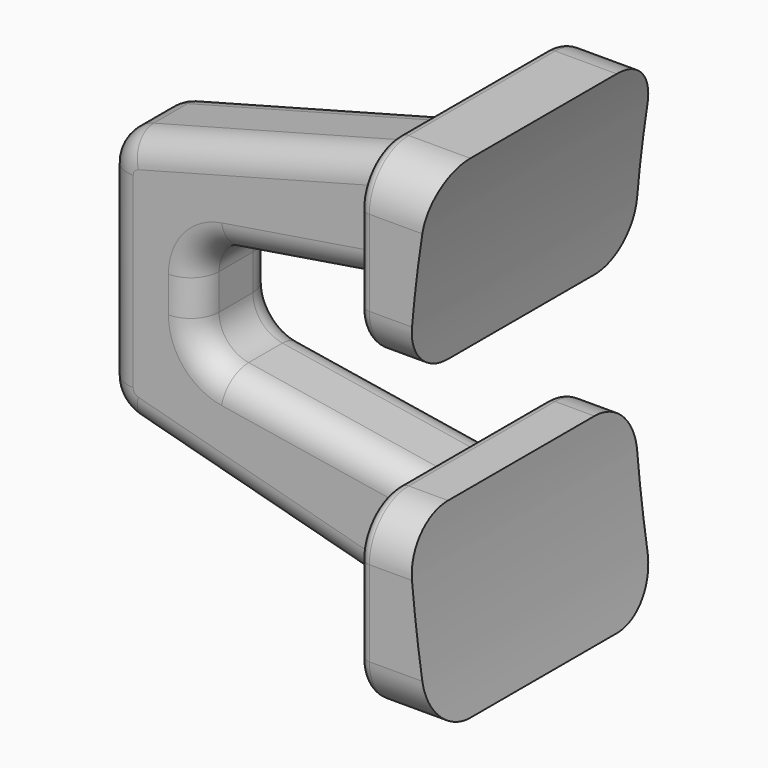
from build123d import *

# Parameters (mm, degrees)
F1_DEPTH = 1.778
F3_DEPTH = 5.08
F4_R     = 1.778
F5_R     = 0.381
F6_R     = 1.27
F7_R     = 1.016
F8_R     = 0.254


# Not quite as in the source:
# - a feature names something its author has since deleted; it is built from what else it names


with BuildPart() as f1:
    # F0 (on Front) → F1 (new body, symmetric)
    with BuildSketch(Plane.XZ):
        with BuildLine():
            Line((-31.496, -8.89), (-28.8890805669, -8.89))
            ThreePointArc((-28.8890805669, -8.89), (-29.4117334596, -5.5835621932), (-29.6945393604, -2.2480385704))
            Line((-29.6945393604, -2.2480385704), (-31.496, -2.2480385704))
            Line((-31.496, -2.2480385704), (-31.496, -3.0988187389))
            Line((-31.496, -3.0988187389), (-39.9942283773, -1.7265919268))
            Line((-39.9942283773, -1.7265919268), (-39.9942283773, 0))
            Line((-39.9942283773, 0), (-39.9942283773, 1.7265919268))
            Line((-39.9942283773, 1.7265919268), (-31.496, 3.0988187389))
            Line((-31.496, 3.0988187389), (-31.496, 2.2480385704))
            Line((-31.496, 2.2480385704), (-29.6945393604, 2.2480385704))
            ThreePointArc((-29.6945393604, 2.2480385704), (-29.4117334596, 5.5835621932), (-28.8890805669, 8.89))
            Line((-28.8890805669, 8.89), (-31.496, 8.89))
            Line((-31.496, 8.89), (-31.496, 7.4847033247))
            Line((-31.496, 7.4847033247), (-43.2962283773, 4.3461126307))
            Line((-43.2962283773, 4.3461126307), (-43.2962283773, 0))
            Line((-43.2962283773, 0), (-43.2962283773, -4.3461126307))
            Line((-43.2962283773, -4.3461126307), (-31.496, -7.4847033247))
            Line((-31.496, -7.4847033247), (-31.496, -8.89))
        make_face()
    extrude(amount=F1_DEPTH, both=True)

    # F2 (on Front) → F3 (join, symmetric)
    with BuildSketch(Plane.XZ):
        with BuildLine():
            Line((-28.8890805669, 8.89), (-31.496, 8.89))
            Line((-31.496, 8.89), (-31.496, 2.2480385704))
            Line((-31.496, 2.2480385704), (-29.6945393604, 2.2480385704))
            ThreePointArc((-29.6945393604, 2.2480385704), (-29.4117334596, 5.5835621932), (-28.8890805669, 8.89))
        make_face()
        with BuildLine():
            Line((-31.496, -2.2480385704), (-31.496, -8.89))
            Line((-31.496, -8.89), (-28.8890805669, -8.89))
            ThreePointArc((-28.8890805669, -8.89), (-29.4117334596, -5.5835621932), (-29.6945393604, -2.2480385704))
            Line((-29.6945393604, -2.2480385704), (-31.496, -2.2480385704))
        make_face()
    extrude(amount=F3_DEPTH, both=True)

    # F4
    f4_edges = [f1.edges().sort_by_distance(p)[0] for p in [
        (-30.19254, -5.08, 8.89),
        (-30.19254, 5.08, 8.89),
        (-30.19254, 5.08, -8.89),
        (-30.19254, -5.08, -8.89),
        (-30.59527, -5.08, -2.248039),
        (-30.59527, -5.08, 2.248039),
        (-30.59527, 5.08, -2.248039),
        (-30.59527, 5.08, 2.248039),
    ]]
    fillet(f4_edges, radius=F4_R)

    # F5
    f5_edges = [f1.edges().sort_by_distance(p)[0] for p in [
        (-31.496, 5.08, 5.569019),
        (-31.496, 4.559236, 8.369236),
        (-31.496, 0, 8.89),
        (-31.496, -5.08, -5.569019),
        (-31.496, -4.559236, -2.768803),
        (-31.496, -4.559236, -8.369236),
        (-31.496, 0, -2.248039),
        (-31.496, 0, -8.89),
        (-31.496, 4.559236, -2.768803),
        (-31.496, 4.559236, -8.369236),
        (-31.496, 5.08, -5.569019),
        (-31.496, 4.559236, 2.768803),
        (-31.496, 0, 2.248039),
        (-31.496, -4.559236, 8.369236),
        (-31.496, -4.559236, 2.768803),
        (-31.496, -5.08, 5.569019),
    ]]
    fillet(f5_edges, radius=F5_R)

    # F6
    f6_edges = [f1.edges().sort_by_distance(p)[0] for p in [
        (-43.296228, 0, -4.346113),
        (-43.296228, 0, 4.346113),
        (-39.994228, 0, 1.726592),
        (-39.994228, 0, -1.726592),
    ]]
    fillet(f6_edges, radius=F6_R)

    # F7
    f7_edges = [f1.edges().sort_by_distance(p)[0] for p in [
        (-36.924335, -1.778, -6.04089),
        (-36.924335, 1.778, -6.04089),
        (-39.994228, -1.778, 0),
        (-35.211338, 1.778, 2.498895),
        (-43.033075, 1.778, -4.143803),
        (-43.296228, 1.778, 0),
        (-35.211338, 1.778, -2.498895),
        (-43.033075, 1.778, 4.143803),
        (-39.691184, 1.778, -1.468556),
        (-36.924335, 1.778, 6.04089),
        (-39.994228, 1.778, 0),
        (-39.691184, 1.778, 1.468556),
        (-43.033075, -1.778, -4.143803),
        (-43.296228, -1.778, 0),
        (-35.211338, -1.778, -2.498895),
        (-43.033075, -1.778, 4.143803),
        (-39.691184, -1.778, -1.468556),
        (-36.924335, -1.778, 6.04089),
        (-39.691184, -1.778, 1.468556),
        (-35.211338, -1.778, 2.498895),
    ]]
    fillet(f7_edges, radius=F7_R)

    # F8
    f8_edges = [f1.edges().sort_by_distance(p)[0] for p in [
        (-31.496, -1.778, -5.280679),
        (-31.496, -1.778, 5.280679),
        (-31.496, 0, -7.484703),
        (-31.496, -1.48042, -7.176778),
        (-31.496, 1.48042, -7.176778),
        (-31.496, 1.778, -5.280679),
        (-31.496, -1.48042, -3.400253),
        (-31.496, 1.48042, -3.400253),
        (-31.496, 0, -3.098819),
        (-31.496, 1.778, 5.280679),
        (-31.496, -1.48042, 3.400253),
        (-31.496, -1.48042, 7.176778),
        (-31.496, 1.48042, 7.176778),
        (-31.496, 1.48042, 3.400253),
        (-31.496, 0, 7.484703),
        (-31.496, 0, 3.098819),
    ]]
    fillet(f8_edges, radius=F8_R)


solid = f1.part
